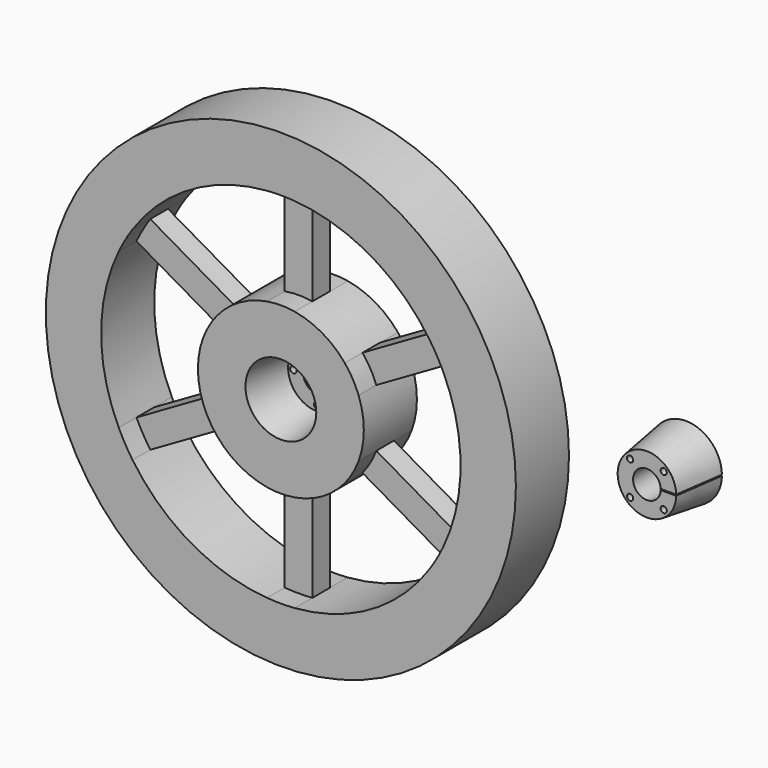
from build123d import *
from build123d import SkipClean  # not in build123d's __all__

# Parameters (mm, degrees)
F0_R        = 107.95
F0_R_2      = 104.775
F0_R_3      = 35.56
F0_R_4      = 6.3627
F1_DEPTH    = 30.48
F3_DEPTH    = 10.16
F6_R        = 13.335
F6_R_2      = 6.3627
F7_DEPTH    = 20.828
F7_FACE_R   = 13.335
F7_FACE_R_2 = 6.3627
F8_DEPTH    = 25.4
F8_TAPER    = -8
F9_R        = 1.4732
F10_DEPTH   = 25.4
F11_R       = 1.4224
F12_DEPTH   = 12.7
F13_R       = 13.4366
F13_R_2     = 1.4224
F13_R_3     = 6.35
F14_DEPTH   = 22.352
F14_TAPER   = -8
F15_DEPTH   = 12.7
F16_DEPTH   = 25.4
F18_DEPTH   = 25.4


# Not quite as in the source:
# - after a boolean that leaves OpenCascade's solid faulty, fix() repairs it
# - a feature of the source that left no trace in its solid (it failed there, or was rolled back) is left out
# - a pattern or mirror of a feature is missing from the dataset's text; its kind, count and spacing are read off the source's solid


with BuildPart() as f1:
    # F0 (on Front) → F1 (new body)
    with BuildSketch(Plane.XZ):
        Circle(F0_R)
        Circle(F0_R_2, mode=Mode.SUBTRACT)
        Circle(F0_R_2)
        with BuildLine():
            Line((-68.103573218, -46.6519647489), (-29.3590686819, -24.2828146254))
            ThreePointArc((-29.3590686819, -24.2828146254), (-19.05, -32.9955678842), (-6.35, -37.5671066227))
            Line((-6.35, -37.5671066227), (-6.35, -82.3054068698))
            ThreePointArc((-6.35, -82.3054068698), (-41.275, -71.4903970824), (-68.103573218, -46.6519647489))
        make_face(mode=Mode.SUBTRACT)
        with BuildLine():
            Line((6.35, -82.3054068698), (6.35, -37.5671066227))
            ThreePointArc((6.35, -37.5671066227), (19.05, -32.9955678842), (29.3590686819, -24.2828146254))
            Line((29.3590686819, -24.2828146254), (68.103573218, -46.6519647489))
            ThreePointArc((68.103573218, -46.6519647489), (41.275, -71.4903970824), (6.35, -82.3054068698))
        make_face(mode=Mode.SUBTRACT)
        with BuildLine():
            Line((74.453573218, -35.6534421209), (35.7090686819, -13.2842919973))
            ThreePointArc((35.7090686819, -13.2842919973), (38.1, 0), (35.7090686819, 13.2842919973))
            Line((35.7090686819, 13.2842919973), (74.453573218, 35.6534421209))
            ThreePointArc((74.453573218, 35.6534421209), (82.55, 0), (74.453573218, -35.6534421209))
        make_face(mode=Mode.SUBTRACT)
        with BuildLine():
            ThreePointArc((-74.453573218, -35.6534421209), (-82.55, 0), (-74.453573218, 35.6534421209))
            Line((-74.453573218, 35.6534421209), (-35.7090686819, 13.2842919973))
            ThreePointArc((-35.7090686819, 13.2842919973), (-38.1, 0), (-35.7090686819, -13.2842919973))
            Line((-35.7090686819, -13.2842919973), (-74.453573218, -35.6534421209))
        make_face(mode=Mode.SUBTRACT)
        with BuildLine():
            Line((-6.35, 82.3054068698), (-6.35, 65.1078820229))
            Line((-6.35, 65.1078820229), (-6.35, 37.5671066227))
            ThreePointArc((-6.35, 37.5671066227), (-19.05, 32.9955678842), (-29.3590686819, 24.2828146254))
            Line((-29.3590686819, 24.2828146254), (-68.103573218, 46.6519647489))
            ThreePointArc((-68.103573218, 46.6519647489), (-41.275, 71.4903970824), (-6.35, 82.3054068698))
        make_face(mode=Mode.SUBTRACT)
        Circle(F0_R_3, mode=Mode.SUBTRACT)
        with BuildLine():
            Line((6.35, 37.5671066227), (6.35, 65.1078820229))
            Line((6.35, 65.1078820229), (6.35, 82.3054068698))
            ThreePointArc((6.35, 82.3054068698), (41.275, 71.4903970824), (68.103573218, 46.6519647489))
            Line((68.103573218, 46.6519647489), (29.3590686819, 24.2828146254))
            ThreePointArc((29.3590686819, 24.2828146254), (19.05, 32.9955678842), (6.35, 37.5671066227))
        make_face(mode=Mode.SUBTRACT)
        Circle(F0_R_3)
        Circle(F0_R_4, mode=Mode.SUBTRACT)
    extrude(amount=F1_DEPTH)

    # F2 (on face) → F3 (cut)
    with BuildSketch(Plane.XZ.offset(30.48)):
        with BuildLine():
            ThreePointArc((-74.453573218, -35.6534421209), (-71.4903970824, -41.275), (-68.103573218, -46.6519647489))
            Line((-68.103573218, -46.6519647489), (-29.3590686819, -24.2828146254))
            ThreePointArc((-29.3590686819, -24.2828146254), (-32.9955678842, -19.05), (-35.7090686819, -13.2842919973))
            Line((-35.7090686819, -13.2842919973), (-74.453573218, -35.6534421209))
        make_face()
        with BuildLine():
            ThreePointArc((-6.35, -82.3054068698), (0, -82.55), (6.35, -82.3054068698))
            Line((6.35, -82.3054068698), (6.35, -37.5671066227))
            ThreePointArc((6.35, -37.5671066227), (0, -38.1), (-6.35, -37.5671066227))
            Line((-6.35, -37.5671066227), (-6.35, -82.3054068698))
        make_face()
        with BuildLine():
            ThreePointArc((68.103573218, -46.6519647489), (71.4903970824, -41.275), (74.453573218, -35.6534421209))
            Line((74.453573218, -35.6534421209), (35.7090686819, -13.2842919973))
            ThreePointArc((35.7090686819, -13.2842919973), (32.9955678842, -19.05), (29.3590686819, -24.2828146254))
            Line((29.3590686819, -24.2828146254), (68.103573218, -46.6519647489))
        make_face()
        with BuildLine():
            Line((35.7090686819, 13.2842919973), (74.453573218, 35.6534421209))
            ThreePointArc((74.453573218, 35.6534421209), (71.4903970824, 41.275), (68.103573218, 46.6519647489))
            Line((68.103573218, 46.6519647489), (29.3590686819, 24.2828146254))
            ThreePointArc((29.3590686819, 24.2828146254), (32.9955678842, 19.05), (35.7090686819, 13.2842919973))
        make_face()
        with BuildLine():
            Line((6.35, 37.5671066227), (6.35, 82.3054068698))
            ThreePointArc((6.35, 82.3054068698), (0, 82.55), (-6.35, 82.3054068698))
            Line((-6.35, 82.3054068698), (-6.35, 37.5671066227))
            ThreePointArc((-6.35, 37.5671066227), (0, 38.1), (6.35, 37.5671066227))
        make_face()
        with BuildLine():
            Line((-29.3590686819, 24.2828146254), (-68.103573218, 46.6519647489))
            ThreePointArc((-68.103573218, 46.6519647489), (-71.4903970824, 41.275), (-74.453573218, 35.6534421209))
            Line((-74.453573218, 35.6534421209), (-35.7090686819, 13.2842919973))
            ThreePointArc((-35.7090686819, 13.2842919973), (-32.9955678842, 19.05), (-29.3590686819, 24.2828146254))
        make_face()
    with SkipClean():  # cleaning this boolean's faces spoils the solid; the shape is the same uncleaned
        f3 = extrude(amount=-F3_DEPTH, mode=Mode.SUBTRACT)

    # F3_copies: F3 across plane
    with SkipClean():  # cleaning this boolean's faces spoils the solid; the shape is the same uncleaned
        add(f3.mirror(Plane.ZX.offset(-15.24)), clean=False, mode=Mode.SUBTRACT)

    # F6 (on face) → F7 (cut)
    with BuildSketch(Plane.XZ.offset(30.48)):
        Circle(F6_R)
        Circle(F6_R_2, mode=Mode.SUBTRACT)
    extrude(amount=-F7_DEPTH, mode=Mode.SUBTRACT)

    add(f1.part.fix(), mode=Mode.REPLACE)

    # F7_face (on face) → F8 (cut)
    with BuildSketch(Plane.XZ.offset(9.652)):
        Circle(F7_FACE_R)
        Circle(F7_FACE_R_2, mode=Mode.SUBTRACT)
    extrude(amount=F8_DEPTH, taper=F8_TAPER, mode=Mode.SUBTRACT)

    # F9 (on face) → F10 (cut)
    with BuildSketch(Plane(origin=(0, 0, 0), x_dir=(-1, 0, 0), z_dir=(0, 1, 0))):
        with Locations((-10.922, 0)):
            Circle(F9_R)
        with Locations((0, 10.922)):
            Circle(F9_R)
        with Locations((0, -10.922)):
            Circle(F9_R)
        with Locations((10.922, 0)):
            Circle(F9_R)
    extrude(amount=-F10_DEPTH, mode=Mode.SUBTRACT)

    # F11 (on face) → F12 (cut)
    with BuildSketch(Plane(origin=(0, 0, 0), x_dir=(-1, 0, 0), z_dir=(0, 1, 0))):
        with Locations((-16.51, 0)):
            Circle(F11_R)
        with Locations((16.51, 0)):
            Circle(F11_R)
    extrude(amount=-F12_DEPTH, mode=Mode.SUBTRACT)


with BuildPart() as f14:
    # F13 (on Front) → F14 (new body)
    with BuildSketch(Plane.XZ):
        with Locations((143.7321156263, 0)):
            Circle(F13_R)
        with Locations((136.0090953622, -7.7230202641)):
            Circle(F13_R_2, mode=Mode.SUBTRACT)
        with Locations((143.7321156263, 0)):
            Circle(F13_R_3, mode=Mode.SUBTRACT)
        with Locations((151.4551358905, -7.7230202641)):
            Circle(F13_R_2, mode=Mode.SUBTRACT)
        with Locations((136.0090953622, 7.7230202641)):
            Circle(F13_R_2, mode=Mode.SUBTRACT)
        with Locations((151.4551358905, 7.7230202641)):
            Circle(F13_R_2, mode=Mode.SUBTRACT)
        with Locations((136.0090953622, 7.7230202641)):
            Circle(F13_R_2)
        with Locations((136.0090953622, -7.7230202641)):
            Circle(F13_R_2)
        with Locations((151.4551358905, -7.7230202641)):
            Circle(F13_R_2)
        with Locations((151.4551358905, 7.7230202641)):
            Circle(F13_R_2)
        with Locations((143.7321156263, 0)):
            Circle(F13_R_3)
    extrude(amount=-F14_DEPTH, taper=F14_TAPER)

    # F13 (on Front) → F15 (cut)
    with BuildSketch(Plane.XZ):
        with Locations((136.0090953622, 7.7230202641)):
            Circle(F13_R_2)
        with Locations((151.4551358905, 7.7230202641)):
            Circle(F13_R_2)
        with Locations((151.4551358905, -7.7230202641)):
            Circle(F13_R_2)
        with Locations((136.0090953622, -7.7230202641)):
            Circle(F13_R_2)
    extrude(amount=-F15_DEPTH, mode=Mode.SUBTRACT)

    # F13 (on Front) → F16 (cut)
    with BuildSketch(Plane.XZ):
        with Locations((143.7321156263, 0)):
            Circle(F13_R_3)
    extrude(amount=-F16_DEPTH, mode=Mode.SUBTRACT)

    # F17 (on face) → F18 (cut)
    with BuildSketch(Plane.XZ):
        with BuildLine():
            ThreePointArc((157.1687156263, 0), (157.1681153703, 0.1270056738), (157.1663146557, 0.254))
            Line((157.1663146557, 0.254), (150.0770335927, 0.254))
            ThreePointArc((150.0770335927, 0.254), (150.0808449908, 0.1270254178), (150.0821156263, 0))
            ThreePointArc((150.0821156263, 0), (150.0808449908, -0.1270254178), (150.0770335927, -0.254))
            Line((150.0770335927, -0.254), (157.1663146557, -0.254))
            ThreePointArc((157.1663146557, -0.254), (157.1681153703, -0.1270056738), (157.1687156263, 0))
        make_face()
        with BuildLine():
            Line((162.7761095905, -0.254), (162.7761095905, 0.254))
            Line((162.7761095905, 0.254), (157.1663146557, 0.254))
            ThreePointArc((157.1663146557, 0.254), (157.1681153703, 0.1270056738), (157.1687156263, 0))
            ThreePointArc((157.1687156263, 0), (157.1681153703, -0.1270056738), (157.1663146557, -0.254))
            Line((157.1663146557, -0.254), (162.7761095905, -0.254))
        make_face()
    extrude(amount=-F18_DEPTH, mode=Mode.SUBTRACT)


solid = Compound([f1.part, f14.part])
